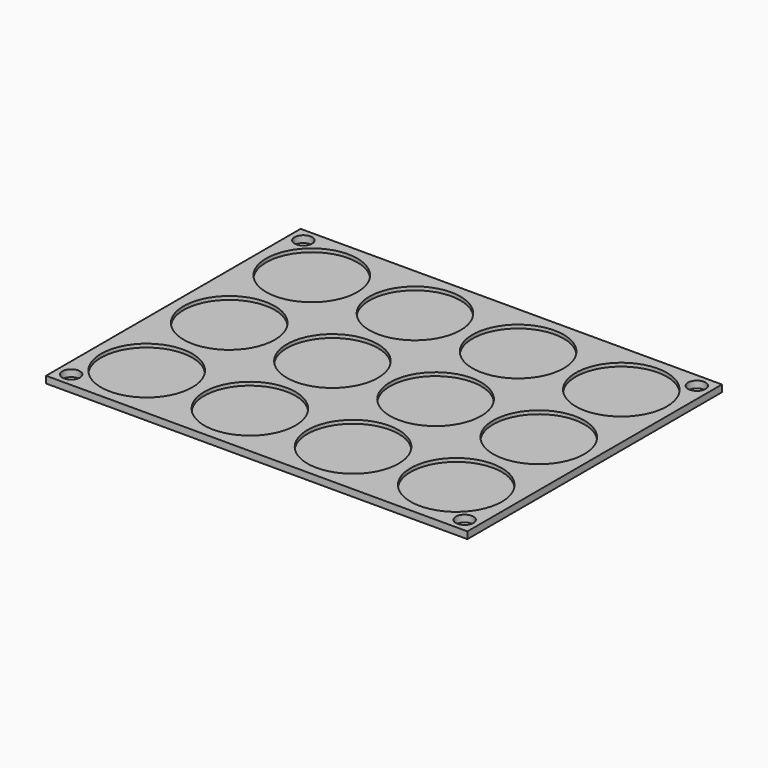
from build123d import *

# Parameters (mm, degrees)
F0_W     = 122.5
F0_H     = 92.5
F0_R     = 13.25
F1_DEPTH = 1
F2_DEPTH = 2
F3_R     = 2.55
F4_DEPTH = 2.001


# Not quite as in the source:
# - a feature names something its author has since deleted; it is built from what else it names


with BuildPart() as f1:
    # F0 (on Top) → F1 (new body)
    with BuildSketch(Plane.XY):
        Rectangle(F0_W, F0_H)
        with Locations((-45, -30)):
            Circle(F0_R, mode=Mode.SUBTRACT)
        with Locations((-15, -30)):
            Circle(F0_R, mode=Mode.SUBTRACT)
        with Locations((15, -30)):
            Circle(F0_R, mode=Mode.SUBTRACT)
        with Locations((45, -30)):
            Circle(F0_R, mode=Mode.SUBTRACT)
        with Locations((-45, 0)):
            Circle(F0_R, mode=Mode.SUBTRACT)
        with Locations((-15, 0)):
            Circle(F0_R, mode=Mode.SUBTRACT)
        with Locations((-45, 30)):
            Circle(F0_R, mode=Mode.SUBTRACT)
        with Locations((-15, 30)):
            Circle(F0_R, mode=Mode.SUBTRACT)
        with Locations((15, 0)):
            Circle(F0_R, mode=Mode.SUBTRACT)
        with Locations((45, 0)):
            Circle(F0_R, mode=Mode.SUBTRACT)
        with Locations((15, 30)):
            Circle(F0_R, mode=Mode.SUBTRACT)
        with Locations((45, 30)):
            Circle(F0_R, mode=Mode.SUBTRACT)
        with Locations((-45, 30)):
            Circle(F0_R)
        with Locations((-15, 30)):
            Circle(F0_R)
        with Locations((15, 30)):
            Circle(F0_R)
        with Locations((45, 30)):
            Circle(F0_R)
        with Locations((45, 0)):
            Circle(F0_R)
        with Locations((-15, 0)):
            Circle(F0_R)
        with Locations((-45, 0)):
            Circle(F0_R)
        with Locations((15, 0)):
            Circle(F0_R)
        with Locations((15, -30)):
            Circle(F0_R)
        with Locations((-15, -30)):
            Circle(F0_R)
        with Locations((-45, -30)):
            Circle(F0_R)
        with Locations((45, -30)):
            Circle(F0_R)
    extrude(amount=F1_DEPTH)

    # F0 (on Top) → F2 (join)
    with BuildSketch(Plane.XY):
        Rectangle(F0_W, F0_H)
        with Locations((-45, -30)):
            Circle(F0_R, mode=Mode.SUBTRACT)
        with Locations((-15, -30)):
            Circle(F0_R, mode=Mode.SUBTRACT)
        with Locations((15, -30)):
            Circle(F0_R, mode=Mode.SUBTRACT)
        with Locations((45, -30)):
            Circle(F0_R, mode=Mode.SUBTRACT)
        with Locations((-45, 0)):
            Circle(F0_R, mode=Mode.SUBTRACT)
        with Locations((-15, 0)):
            Circle(F0_R, mode=Mode.SUBTRACT)
        with Locations((-45, 30)):
            Circle(F0_R, mode=Mode.SUBTRACT)
        with Locations((-15, 30)):
            Circle(F0_R, mode=Mode.SUBTRACT)
        with Locations((15, 0)):
            Circle(F0_R, mode=Mode.SUBTRACT)
        with Locations((45, 0)):
            Circle(F0_R, mode=Mode.SUBTRACT)
        with Locations((15, 30)):
            Circle(F0_R, mode=Mode.SUBTRACT)
        with Locations((45, 30)):
            Circle(F0_R, mode=Mode.SUBTRACT)
    extrude(amount=F2_DEPTH)

    # F3 (on face) → F4 (cut, through all)
    with BuildSketch(Plane.XY.offset(2)):
        with Locations((-57.2, 42.2)):
            Circle(F3_R)
        with Locations((57.2, 42.2)):
            Circle(F3_R)
        with Locations((-57.2, -42.2)):
            Circle(F3_R)
        with Locations((57.2, -42.2)):
            Circle(F3_R)
    extrude(amount=-F4_DEPTH, mode=Mode.SUBTRACT)


solid = f1.part
